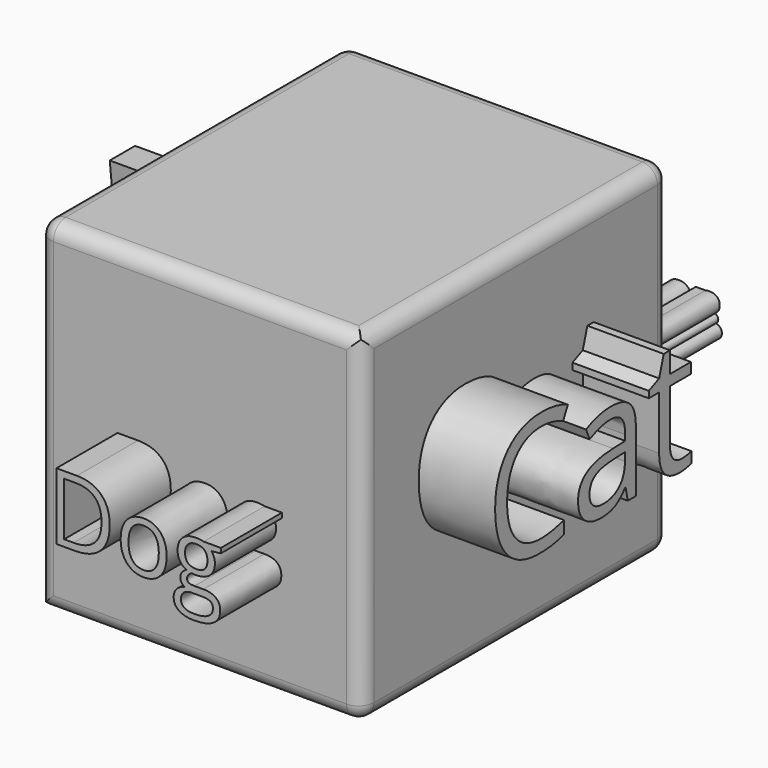
from build123d import *

# Parameters (mm, degrees)
F0_W          = 107.6527945697
F0_H          = 113.820925355
F1_DEPTH      = 128.016
F2_R          = 5.08
F3_T1_DEPTH   = 117.856
F3_T3_DEPTH   = 110.1927945697
F3_T5_DEPTH   = 116.360925355
F3_S9_W       = 5.1816
F3_S9_H       = 5.1816
F3_T10_DEPTH  = 5.1816
F3_S15_W      = 5.1816
F3_S15_H      = 5.1816
F3_T16_DEPTH  = 5.1816
F4_TEXT_SIZE  = 31.0987783855
F5_DEPTH      = 25.4
F6_TEXT_SIZE  = 55.9915633251
F7_DEPTH      = 25.4
F8_TEXT_SIZE  = 111.3354797579
F9_DEPTH      = 25.4
F10_TEXT_SIZE = 17.2285517461
F11_DEPTH     = 25.4


# Not quite as in the source:
# - a fillet or chamfer that OpenCascade refuses, or shapes differently, is made with other operations: its cross-section is extruded or revolved along the edge and cut away or added
# - Text() gives the source's letters only with a copy of the font that has no kerning and outlines rounded to 1/6400 em; it was checked with that copy


with BuildPart() as f1:
    # F0 (on Front) → F1 (new body)
    with BuildSketch(Plane.XZ):
        with Locations((-2.2959131747, -2.958688885)):
            Rectangle(F0_W, F0_H)
    extrude(amount=F1_DEPTH)

    # F2
    f2_edges = [f1.edges().sort_by_distance(p)[0] for p in [
        (-56.12231, -64.008, -59.869152),
        (-2.295913, 0, 53.951774),
        (-56.12231, 0, -2.958689),
        (-2.295913, 0, -59.869152),
        (51.530484, 0, -2.958689),
        (51.530484, -64.008, 53.951774),
        (-56.12231, -64.008, 53.951774),
        (-2.295913, -128.016, 53.951774),
        (-56.12231, -128.016, -2.958689),
    ]]
    fillet(f2_edges, radius=F2_R)

    # F3: fillet of radius 5.08 on 13 edges, made by hand

    # F3_s2 → F3_t1 (cut)
    with BuildSketch(Plane.XZ.offset(5.08)):
        with BuildLine():
            ThreePointArc((51.5304841101, -54.7891515625), (50.0425865585, -58.3812540109), (46.4504841101, -59.8691515625))
            Line((46.4504841101, -59.8691515625), (51.5304841101, -59.8691515625))
            Line((51.5304841101, -59.8691515625), (51.5304841101, -54.7891515625))
        make_face()
    extrude(amount=F3_T1_DEPTH, mode=Mode.SUBTRACT)

    # F3_s4 → F3_t3 (cut)
    with BuildSketch(Plane.YZ.offset(-63.7423104596)):
        with BuildLine():
            ThreePointArc((-128.016, -54.7891515625), (-126.5281024484, -58.3812540109), (-122.936, -59.8691515625))
            Line((-122.936, -59.8691515625), (-128.016, -59.8691515625))
            Line((-128.016, -59.8691515625), (-128.016, -54.7891515625))
        make_face()
    extrude(amount=F3_T3_DEPTH, mode=Mode.SUBTRACT)

    # F3_s6 → F3_t5 (cut)
    with BuildSketch(Plane.XY.offset(-54.7891515625)):
        with BuildLine():
            ThreePointArc((51.5304841101, -122.936), (50.0425865585, -126.5281024484), (46.4504841101, -128.016))
            Line((46.4504841101, -128.016), (51.5304841101, -128.016))
            Line((51.5304841101, -128.016), (51.5304841101, -122.936))
        make_face()
    extrude(amount=F3_T5_DEPTH, mode=Mode.SUBTRACT)


with BuildPart() as f3_tool8:
    # F3_s9 → F3_t10 (new body)
    with BuildSketch(Plane.YZ.offset(46.4504841101)):
        with Locations((-2.4892, -57.3799515625)):
            Rectangle(F3_S9_W, F3_S9_H)
    extrude(amount=F3_T10_DEPTH)

    # F3_s11 → F3_t12 (revolve, cut)
    with BuildSketch(Plane(origin=(46.4504841101, -5.08, -54.7891515625), x_dir=(0, -0.7071067812, 0.7071067812), z_dir=(0, 0.7071067812, 0.7071067812))):
        with BuildLine():
            ThreePointArc((0, -5.08), (5.08, 0), (0, 5.08))
            Line((0, 5.08), (0, -5.08))
        make_face()
    revolve(axis=Axis((46.4504841101, -5.08, -54.7891515625), (1, 0, 0)), mode=Mode.SUBTRACT)


with BuildPart() as f1_1:
    add(f1.part)

    # F3_t7: cut F3_tool8
    add(f3_tool8.part, mode=Mode.SUBTRACT)


with BuildPart() as f3_tool14:
    # F3_s15 → F3_t16 (new body)
    with BuildSketch(Plane.YZ.offset(46.4504841101)):
        with Locations((-125.5268, -57.3799515625)):
            Rectangle(F3_S15_W, F3_S15_H)
    extrude(amount=F3_T16_DEPTH)

    # F3_s17 → F3_t18 (revolve, cut)
    with BuildSketch(Plane(origin=(46.4504841101, -122.936, -54.7891515625), x_dir=(0, 0.7071067812, 0.7071067812), z_dir=(0, 0.7071067812, -0.7071067812))):
        with BuildLine():
            ThreePointArc((0, -5.08), (5.08, 0), (0, 5.08))
            Line((0, 5.08), (0, -5.08))
        make_face()
    revolve(axis=Axis((46.4504841101, -122.936, -54.7891515625), (1, 0, 0)), mode=Mode.SUBTRACT)


with BuildPart() as f1_2:
    add(f1_1.part)

    # F3_t13: cut F3_tool14
    add(f3_tool14.part, mode=Mode.SUBTRACT)

    # F4 (on face) → F5 (join)
    with BuildSketch(Plane.XZ.offset(128.016)):
        with Locations((-32.7727355228, -22.3911204375)):
            Text('Dog', F4_TEXT_SIZE, font='Open Sans', text_align=(TextAlign.LEFT, TextAlign.BOTTOM))
    extrude(amount=F5_DEPTH)

    # F6 (on face) → F7 (join)
    with BuildSketch(Plane.YZ.offset(51.5304841101)):
        with Locations((-107.7337143943, -17.4104981124)):
            Text('Cat', F6_TEXT_SIZE, font='Open Sans', text_align=(TextAlign.LEFT, TextAlign.BOTTOM))
    extrude(amount=F7_DEPTH)

    # F8 (on face) → F9 (join)
    with BuildSketch(Plane(origin=(-56.1223104596, 0, 0), x_dir=(0, -1, 0), z_dir=(-1, 0, 0))):
        with Locations((30.7753421366, -46.8545109034)):
            Text('*', F8_TEXT_SIZE, font='Open Sans', text_align=(TextAlign.LEFT, TextAlign.BOTTOM))
    extrude(amount=F9_DEPTH)

    # F10 (on face) → F11 (join)
    with BuildSketch(Plane(origin=(0, 0, 0), x_dir=(-1, 0, 0), z_dir=(0, 1, 0))):
        with Locations((-48.9259891719, -6.3369688197)):
            Text('go to college', F10_TEXT_SIZE, font='Open Sans', text_align=(TextAlign.LEFT, TextAlign.BOTTOM))
    extrude(amount=F11_DEPTH)


solid = f1_2.part
